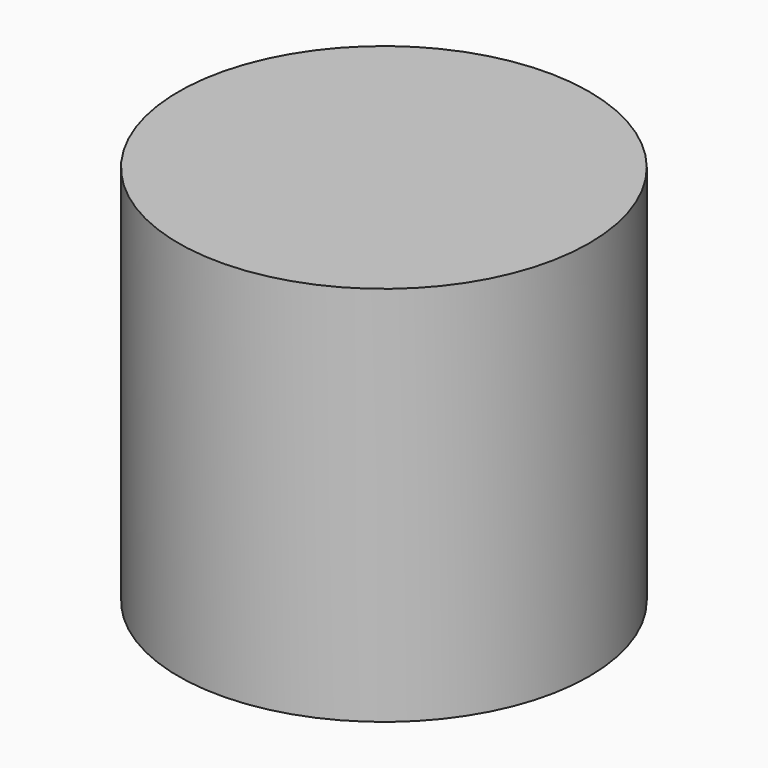
from build123d import *

# Parameters (mm, degrees)
F0_R     = 3.5
F1_DEPTH = 10
F2_T     = -1.5


# Not quite as in the source:
# - a fillet or chamfer that OpenCascade refuses, or shapes differently, is made with other operations: its cross-section is extruded or revolved along the edge and cut away or added


with BuildPart() as f1:
    # F0 (on Top) → F1 (new body)
    with BuildSketch(Plane.XY):
        with Locations((-2.5134360774, -2.4357009433)):
            Circle(F0_R)
    extrude(amount=F1_DEPTH)

    # F2
    f2_openings = [f1.faces().sort_by_distance(p)[0] for p in [
        (-2.513436, -2.435701, 0),
    ]]
    offset(amount=F2_T, openings=f2_openings)

    # F3: chamfer of 5 on 1 edges, made by hand

    # F3_s1 → F3_t2 (revolve, cut)
    with BuildSketch(Plane.XZ.offset(2.4357009433)):
        Polygon((4.4865639226, 0), (-0.5134360774, 5), (-0.5134360774, 0), align=None)
    revolve(axis=Axis((-2.5134360774, -2.4357009433, 0), (0, 0, 1)), mode=Mode.SUBTRACT)


solid = f1.part
